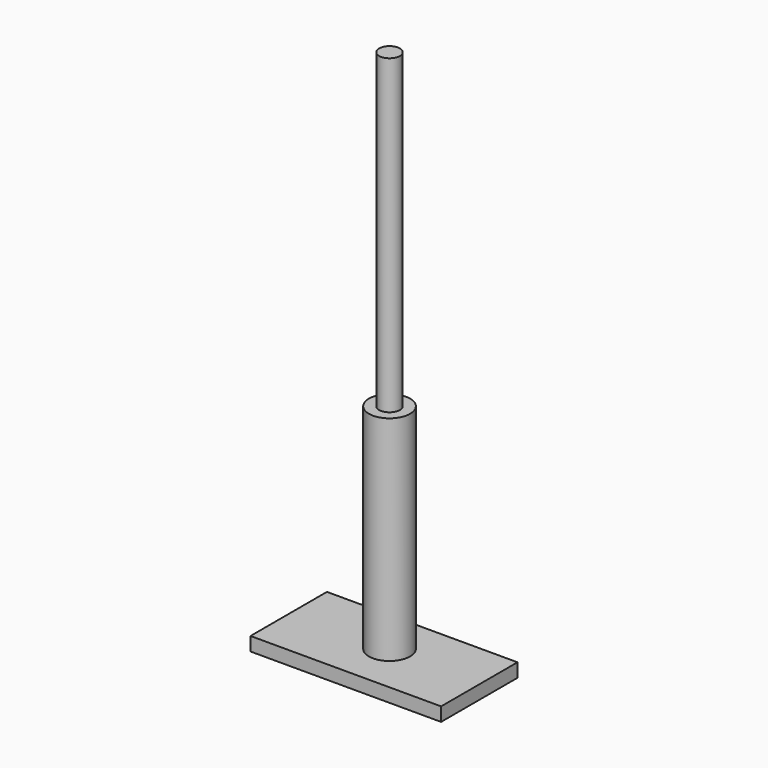
from build123d import *

# Parameters (mm, degrees)
F0_W     = 88.395819068
F0_H     = 44.2917048931
F1_DEPTH = 6.35
F2_R     = 9.5460938565
F3_DEPTH = 99.0852161
F4_R     = 4.7953323776
F5_DEPTH = 144.5512078


# Not quite as in the source:
# - an extrude ends at something that could not be found from the text; its depth is read off the source's solid


with BuildPart() as f1:
    # F0 (on Top) → F1 (new body)
    with BuildSketch(Plane.XY):
        with Locations((-1.4388076961, -22.1458524466)):
            Rectangle(F0_W, F0_H)
    extrude(amount=F1_DEPTH)

    # F2 (on face) → F3 (join, through all)
    with BuildSketch(Plane.XY.offset(6.35)):
        with Locations((0, -20.7415707409)):
            Circle(F2_R)
    extrude(amount=F3_DEPTH)

    # F4 (on face) → F5 (join, through all)
    with BuildSketch(Plane.XY.offset(105.4352161291)):
        with Locations((0, -20.7415707409)):
            Circle(F4_R)
    extrude(amount=F5_DEPTH)


solid = f1.part
